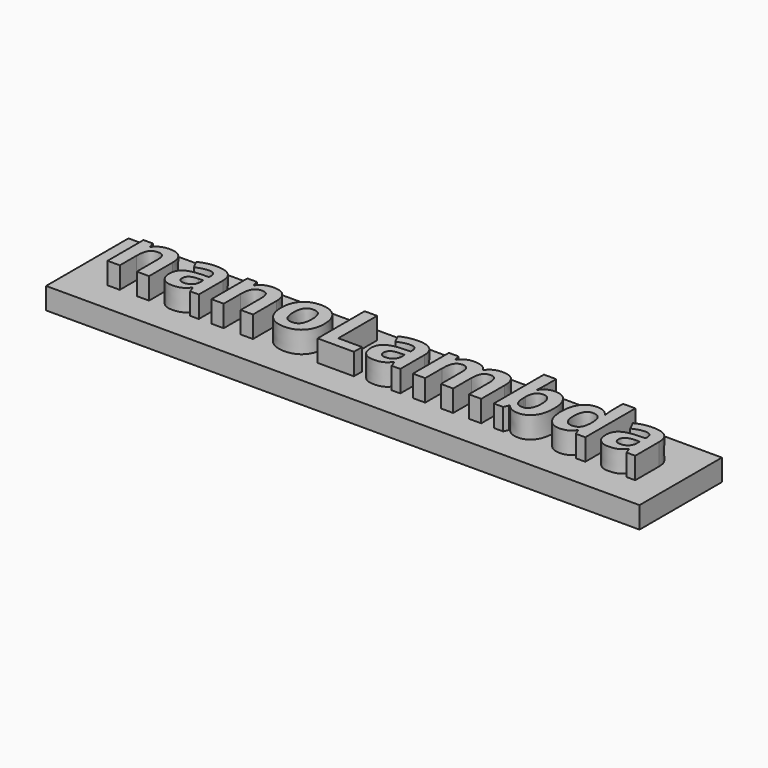
from build123d import *

# Parameters (mm, degrees)
F0_TEXT_SIZE = 7.6361380232
F1_DEPTH     = 2
F2_W         = 55
F2_H         = 9.5470174443
F3_DEPTH     = 2


# Not quite as in the source:
# - Text() gives the source's letters only with a copy of the font that has no kerning and outlines rounded to 1/6400 em; it was checked with that copy


with BuildPart() as f1:
    # F0 (on Top) → F1 (new body)
    with BuildSketch(Plane.XY):
        with Locations((-8.1293990153, -2.8592645112)):
            Text('nanoLambda', F0_TEXT_SIZE, font='Open Sans', font_style=FontStyle.BOLD, text_align=(TextAlign.LEFT, TextAlign.BOTTOM))
    extrude(amount=F1_DEPTH)


with BuildPart() as f3:
    # F2 (on Top) → F3 (new body)
    with BuildSketch(Plane.XY):
        with Locations((16.5548850782, -0.9395279922)):
            Rectangle(F2_W, F2_H)
    extrude(amount=-F3_DEPTH)


solid = Compound([f1.part, f3.part])
